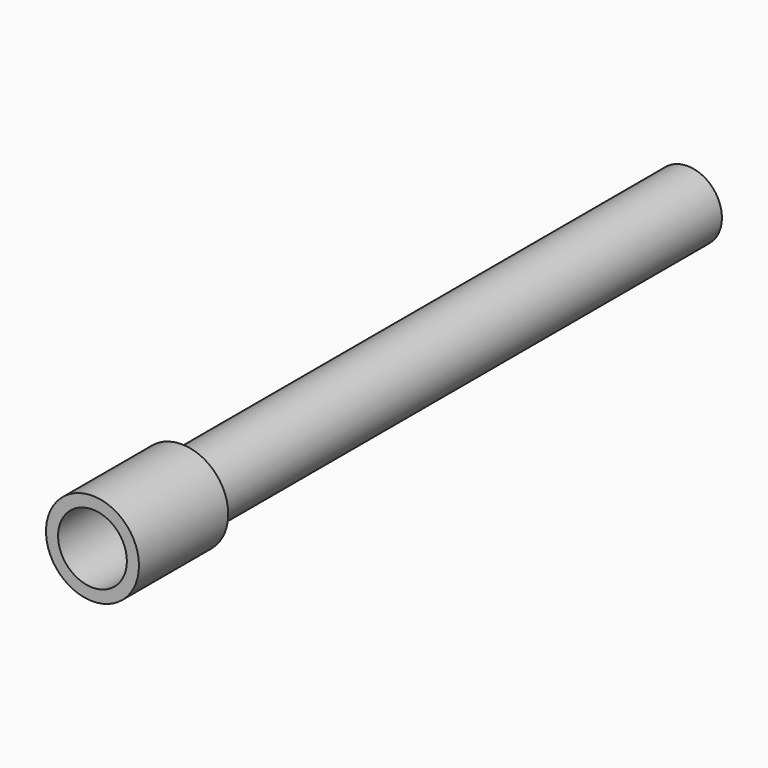
from build123d import *

# Parameters (mm, degrees)
F0_R     = 4.699
F1_DEPTH = 88.9
F2_R     = 6.35
F2_R_2   = 4.699
F3_DEPTH = 12.7
F4_DEPTH = 2.54


with BuildPart() as f1:
    # F0 (on Front) → F1 (new body)
    with BuildSketch(Plane.XZ):
        Circle(F0_R)
    extrude(amount=F1_DEPTH)

    # F2 (on face) → F3 (join)
    with BuildSketch(Plane.XZ.offset(88.9)):
        Circle(F2_R)
        Circle(F2_R_2, mode=Mode.SUBTRACT)
    extrude(amount=F3_DEPTH)

    # F4 (add): a face of the model
    f4_faces = [f1.faces().sort_by_distance(p)[0] for p in [
        (-6.1703948776, -88.9, 0),
    ]]
    extrude(f4_faces, amount=F4_DEPTH)


solid = f1.part
